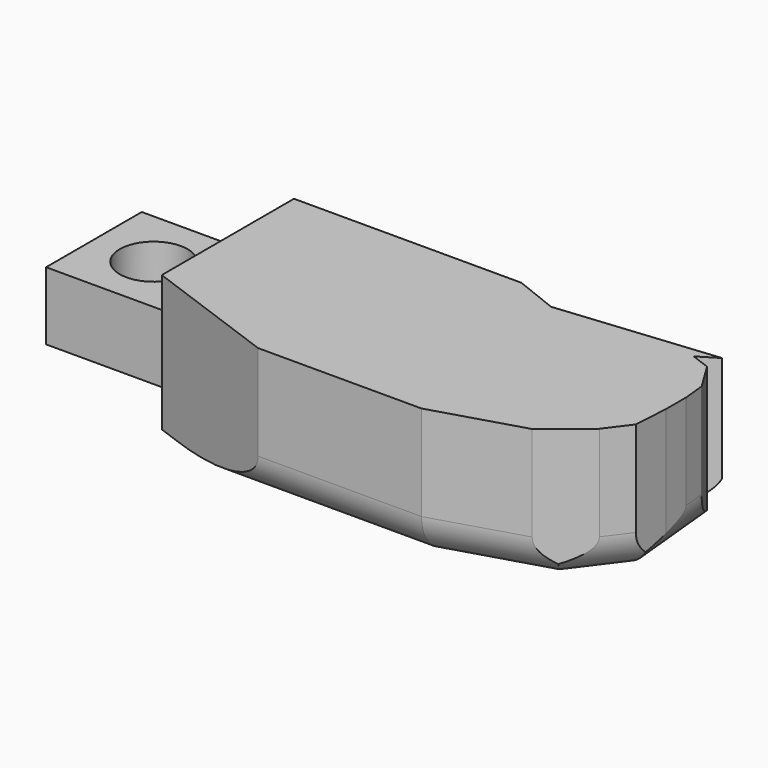
from build123d import *

# Parameters (mm, degrees)
F0_R        = 2.5
F1_DEPTH    = 10
F2_W        = 8.8
F2_H        = 8.8
F2_R        = 2.5
F3_DEPTH    = 2.5
F4_W        = 8.8
F4_H        = 8.8
F4_R        = 2.5
F5_DEPTH    = 2.5
F6_T1_DEPTH = 52.7272001401
F6_T3_DEPTH = 37.6344553761
F6_T5_DEPTH = 42.8447953281
F6_T7_DEPTH = 58.0308217405
F6_T9_DEPTH = 38.1595084339
F7_T1_DEPTH = 58.883894651


# Not quite as in the source:
# - a fillet or chamfer that OpenCascade refuses, or shapes differently, is made with other operations: its cross-section is extruded or revolved along the edge and cut away or added


with BuildPart() as f1:
    # F0 (on Top) → F1 (new body)
    with BuildSketch(Plane.XY):
        Polygon((10.7213496009, 14.3520427298), (0, 14.3520427298), (-6.0058505391, 14.3520427298), (-6.0058505391, 11.3520427298), (-14.8058505391, 11.3520427298), (-14.8058505391, 2.5520427298), (-6.0058505391, 2.5520427298), (-6.0058505391, -1.4479572702), (0, -1.4479572702), (16.0249712014, -1.4479572702), (22.5786776848, 0.5269235903), (25.5761091025, 2.9657761595), (26.8709543148, 4.6940274585), (27.0316003021, 7.267983998), (27.0316003021, 9.1232445721), (26.8709543148, 10.7497860696), (25.5761091025, 12.8667177236), (24.1809434093, 13.3803505253), (25.5761091025, 14.2337194165), (13.9262006316, 13.0831117922), align=None)
        with Locations((-10.4058505391, 6.9520427298)):
            Circle(F0_R, mode=Mode.SUBTRACT)
    extrude(amount=F1_DEPTH)

    # F2 (on face) → F3 (cut)
    with BuildSketch(Plane.XY.offset(10)):
        with Locations((-10.4058505391, 6.9520427298)):
            Rectangle(F2_W, F2_H)
        with Locations((-10.4058505391, 6.9520427298)):
            Circle(F2_R, mode=Mode.SUBTRACT)
    extrude(amount=-F3_DEPTH, mode=Mode.SUBTRACT)

    # F4 (on face) → F5 (cut)
    with BuildSketch(Plane(origin=(0, 0, 0), x_dir=(1, 0, 0), z_dir=(0, 0, -1))):
        with Locations((-10.4058505391, -6.9520427298)):
            Rectangle(F4_W, F4_H)
        with Locations((-10.4058505391, -6.9520427298)):
            Circle(F4_R, mode=Mode.SUBTRACT)
    extrude(amount=-F5_DEPTH, mode=Mode.SUBTRACT)

    # F6: fillet of radius 3 on 5 edges, made by hand

    # F6_s2 → F6_t1 (cut)
    with BuildSketch(Plane.YZ.offset(-24.0058505391)):
        with BuildLine():
            ThreePointArc((14.3520427298, 3), (13.4733630734, 0.8786796564), (11.3520427298, 0))
            Line((11.3520427298, 0), (11.3520427298, -0.06))
            Line((11.3520427298, -0.06), (14.4120427298, -0.06))
            Line((14.4120427298, -0.06), (14.4120427298, 3))
            Line((14.4120427298, 3), (14.3520427298, 3))
        make_face()
    extrude(amount=F6_T1_DEPTH, mode=Mode.SUBTRACT)

    # F6_s4 → F6_t3 (cut)
    with BuildSketch(Plane(origin=(1.1379480439, -11.5217301503, 0), x_dir=(0, 0, 1), z_dir=(-0.0982871663, 0.9951580944, 0))):
        with BuildLine():
            ThreePointArc((0, 24.7974137027), (0.8786796564, 26.9187340462), (3, 27.7974137027))
            Line((3, 27.7974137027), (3, 27.8574137027))
            Line((3, 27.8574137027), (-0.06, 27.8574137027))
            Line((-0.06, 27.8574137027), (-0.06, 24.7974137027))
            Line((-0.06, 24.7974137027), (0, 24.7974137027))
        make_face()
    extrude(amount=F6_T3_DEPTH, mode=Mode.SUBTRACT)

    # F6_s6 → F6_t5 (cut)
    with BuildSketch(Plane(origin=(-2.9435517348, -0.8870040179, 0), x_dir=(0, 0, 1), z_dir=(0.9574729658, 0.2885229968, 0))):
        with BuildLine():
            ThreePointArc((0, 3.0099526564), (0.8786796564, 5.131273), (3, 6.0099526564))
            Line((3, 6.0099526564), (3, 6.0699526564))
            Line((3, 6.0699526564), (-0.06, 6.0699526564))
            Line((-0.06, 6.0699526564), (-0.06, 3.0099526564))
            Line((-0.06, 3.0099526564), (0, 3.0099526564))
        make_face()
    extrude(amount=F6_T5_DEPTH, mode=Mode.SUBTRACT)

    # F6_s8 → F6_t7 (cut)
    with BuildSketch(Plane.YZ.offset(-24.0058505391)):
        with BuildLine():
            ThreePointArc((1.5520427298, 0), (-0.5692776137, 0.8786796564), (-1.4479572702, 3))
            Line((-1.4479572702, 3), (-1.5079572702, 3))
            Line((-1.5079572702, 3), (-1.5079572702, -0.06))
            Line((-1.5079572702, -0.06), (1.5520427298, -0.06))
            Line((1.5520427298, -0.06), (1.5520427298, 0))
        make_face()
    extrude(amount=F6_T7_DEPTH, mode=Mode.SUBTRACT)

    # F6_s10 → F6_t9 (cut)
    with BuildSketch(Plane(origin=(-0.1744913342, -0.2328964668, 0), x_dir=(0, 0, 1), z_dir=(0.5996018316, 0.8002984715, 0))):
        with BuildLine():
            ThreePointArc((0, 15.6902362056), (0.8786796564, 17.8115565491), (3, 18.6902362056))
            Line((3, 18.6902362056), (3, 18.7502362056))
            Line((3, 18.7502362056), (-0.06, 18.7502362056))
            Line((-0.06, 18.7502362056), (-0.06, 15.6902362056))
            Line((-0.06, 15.6902362056), (0, 15.6902362056))
        make_face()
    extrude(amount=F6_T9_DEPTH, mode=Mode.SUBTRACT)

    # F7: chamfer of 10 x 3.6397023427 on 1 edges, made by hand

    # F7_s2 → F7_t1 (cut)
    with BuildSketch(Plane.XY.offset(-22.9419473255)):
        Polygon((-6.0058505391, 2.1917450725), (3.9941494609, -1.4479572702), (-6.0058505391, -1.4479572702), align=None)
    extrude(amount=F7_T1_DEPTH, mode=Mode.SUBTRACT)


solid = f1.part
